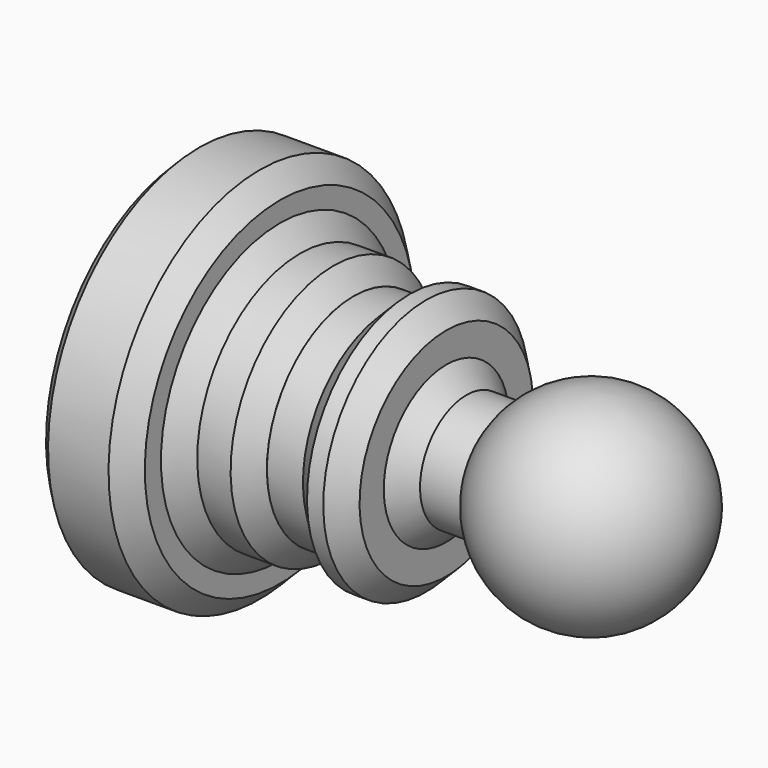
from build123d import *

# Parameters (mm, degrees)
F2_SIZE = 0.508
F3_SIZE = 0.254


with BuildPart() as f1:
    # F0 (on Front) → F1 (revolve)
    with BuildSketch(Plane.XZ):
        with BuildLine():
            Line((-12.7, 0), (0, 0))
            ThreePointArc((0, 0), (-1.81176033, 2.4603689383), (-4.699, 1.4605))
            Line((-4.699, 1.4605), (-6.223, 1.4605))
            Line((-6.223, 1.4605), (-6.223, 3.2385))
            Line((-6.223, 3.2385), (-7.6489057392, 3.2385))
            Line((-7.6489057392, 3.2385), (-7.6489057392, 2.7284773532))
            Line((-7.6489057392, 2.7284773532), (-8.558110334, 2.7284773532))
            Line((-8.558110334, 2.7284773532), (-8.558110334, 3.2385))
            Line((-8.558110334, 3.2385), (-10.414, 3.2385))
            Line((-10.414, 3.2385), (-10.414, 4.7625))
            Line((-10.414, 4.7625), (-12.7, 4.7625))
            Line((-12.7, 4.7625), (-12.7, 0))
        make_face()
    revolve(axis=Axis((-6.35, 0, 0), (-1, 0, 0)))

    # F2
    f2_edges = [f1.edges().sort_by_distance(p)[0] for p in [
        (-10.414, 0, -4.7625),
        (-7.648906, 0, -3.2385),
        (-6.223, 0, -1.4605),
        (-6.223, 0, -3.2385),
        (-8.55811, 0, -3.2385),
        (-10.414, 0, -3.2385),
    ]]
    chamfer(f2_edges, length=F2_SIZE)

    # F3
    f3_edges = [f1.edges().sort_by_distance(p)[0] for p in [
        (-12.7, 0, -4.7625),
    ]]
    chamfer(f3_edges, length=F3_SIZE)


solid = f1.part
